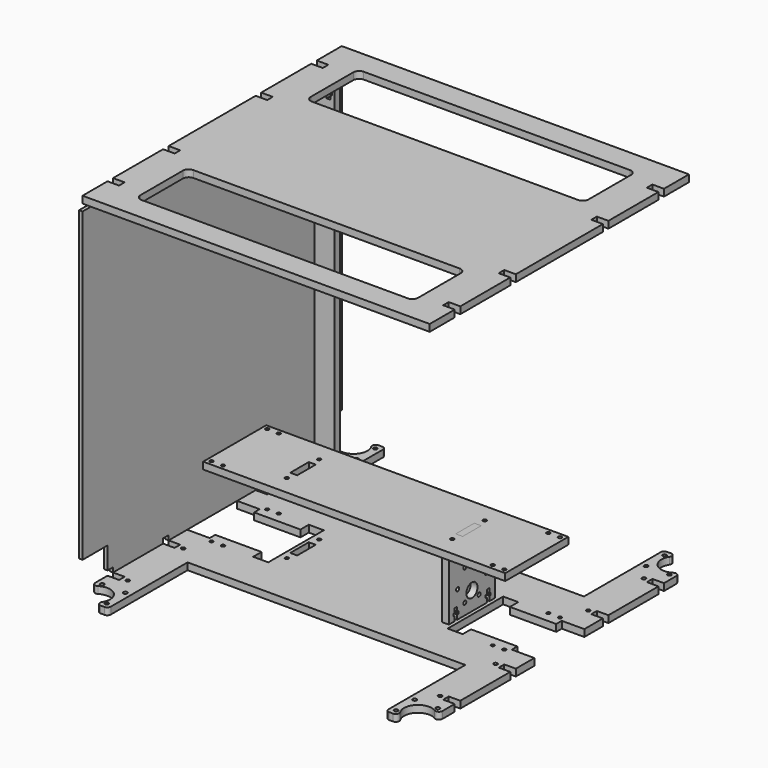
from build123d import *

# Parameters (mm, degrees)
F0_R         = 1.5
F0_W         = 6
F0_H         = 20
F1_DEPTH     = 6
F2_D         = 3
F3_W         = 6
F3_H         = 50
F4_DEPTH     = 55
F5_W         = 6
F5_H         = 20
F6_DEPTH     = 6
F7_R         = 6
F7_R_2       = 1.65
F8_DEPTH     = 6
F10_DEPTH    = 6
F11_W        = 6
F11_H        = 20
F12_DEPTH    = 6
F13_W        = 261
F13_H        = 68.1
F13_R        = 1.5
F13_W_2      = 6
F13_H_2      = 20
F14_DEPTH    = 6
F16_DEPTH    = 6
F17_W        = 10
F17_H        = 6
F19_DEPTH    = 6.001
F20_R        = 3
F21_D        = 3.3
F21_ON_F17_D = 3.3
F23_DEPTH    = 6
F25_DEPTH    = 3
F26_W        = 240
F26_H        = 55.95
F27_DEPTH    = 6
F28_R        = 5


with BuildPart() as f1:
    # F0 (on Top) → F1 (new body)
    with BuildSketch(Plane.XY):
        Polygon((150, 27), (150, 34.05), (-150, 34.05), (-150, 27), (-130.5, 27), (-130.5, 21), (-90.5, 21), (-90.5, 30), (-77.5, 30), (-77.5, -30), (-90.5, -30), (-90.5, -21), (-130.5, -21), (-130.5, -27), (-150, -27), (-150, -34.05), (150, -34.05), (150, -27), (130.5, -27), (130.5, -21), (90.5, -21), (90.5, -30), (77.5, -30), (77.5, 30), (90.5, 30), (90.5, 21), (130.5, 21), (130.5, 27), align=None)
        with Locations((-71.5, -17.5)):
            Circle(F0_R, mode=Mode.SUBTRACT)
        with Locations((71.5, -17.5)):
            Circle(F0_R, mode=Mode.SUBTRACT)
        with Locations((-71.5, 0)):
            Rectangle(F0_W, F0_H, mode=Mode.SUBTRACT)
        with Locations((-71.5, 17.5)):
            Circle(F0_R, mode=Mode.SUBTRACT)
        with Locations((71.5, 0)):
            Rectangle(F0_W, F0_H, mode=Mode.SUBTRACT)
        with Locations((71.5, 17.5)):
            Circle(F0_R, mode=Mode.SUBTRACT)
    extrude(amount=F1_DEPTH)

    # F2 (through all)
    with Locations(Plane(origin=(0, 0, 0), x_dir=(1, 0, 0), z_dir=(0, 0, -1))):
        with Locations((126.5, 30.05), (116.5, 30.05), (126.5, -30.05), (116.5, -30.05), (-116.5, 30.05), (-126.5, 30.05), (-116.5, -30.05), (-126.5, -30.05)):
            Hole(F2_D / 2)

    # F15 (on face) → F16 (join)
    with BuildSketch(Plane.XY.offset(6)):
        Polygon((-150, 150), (-150, 34.05), (0, 34.05), (150, 34.05), (150, 150), (120, 150), (120, 64.05), (0, 64.05), (-120, 64.05), (-120, 150), align=None)
        Polygon((0, -34.05), (-150, -34.05), (-150, -150), (-120, -150), (-120, -64.05), (0, -64.05), (120, -64.05), (120, -150), (150, -150), (150, -34.05), align=None)
    extrude(amount=-F16_DEPTH)

    # F17 (on face) → F19 (cut, through all)
    with BuildSketch(Plane.XY.offset(6)):
        with BuildLine():
            Line((-150, -150), (-134.2041684767, -150))
            ThreePointArc((-134.2041684767, -150), (-130.5147186258, -130.5147186258), (-150, -134.2041684767))
            Line((-150, -134.2041684767), (-150, -150))
        make_face()
        with BuildLine():
            Line((134.2041684767, -150), (150, -150))
            Line((150, -150), (150, -134.2041684767))
            ThreePointArc((150, -134.2041684767), (130.5147186258, -130.5147186258), (134.2041684767, -150))
        make_face()
        with BuildLine():
            Line((150, 150), (134.2041684767, 150))
            ThreePointArc((134.2041684767, 150), (130.5147186258, 130.5147186258), (150, 134.2041684767))
            Line((150, 134.2041684767), (150, 150))
        make_face()
        with BuildLine():
            ThreePointArc((-150, 134.2041684767), (-130.5147186258, 130.5147186258), (-134.2041684767, 150))
            Line((-134.2041684767, 150), (-150, 150))
            Line((-150, 150), (-150, 134.2041684767))
        make_face()
        with Locations((-145, 110)):
            Rectangle(F17_W, F17_H)
        with Locations((-145, 50)):
            Rectangle(F17_W, F17_H)
        with Locations((145, 50)):
            Rectangle(F17_W, F17_H)
        with Locations((145, 110)):
            Rectangle(F17_W, F17_H)
        with Locations((145, -110)):
            Rectangle(F17_W, F17_H)
        with Locations((-145, -50)):
            Rectangle(F17_W, F17_H)
        with Locations((145, -50)):
            Rectangle(F17_W, F17_H)
        with Locations((-145, -110)):
            Rectangle(F17_W, F17_H)
    extrude(amount=-F19_DEPTH, mode=Mode.SUBTRACT)

    # F20
    f20_edges = [f1.edges().sort_by_distance(p)[0] for p in [
        (-134.204168, -150, 3),
        (-150, -134.204168, 3),
        (-120, -150, 3),
        (120, -150, 3),
        (134.204168, -150, 3),
        (150, -134.204168, 3),
        (150, 134.204168, 3),
        (134.204168, 150, 3),
        (120, 150, 3),
        (-120, 150, 3),
        (-134.204168, 150, 3),
        (-150, 134.204168, 3),
    ]]
    fillet(f20_edges, radius=F20_R)

    # F21 (through all)
    with Locations(Plane.XY.offset(6)):
        with Locations((-145, 125), (-125, 145), (-125, 125), (145, 125), (125, 125), (125, 145), (-145, -125), (-125, -125), (-125, -145), (125, -145), (145, -125), (125, -125)):
            Hole(F21_D / 2)

    # F21 on F17 (through all)
    with Locations(Plane.XY.offset(6)):
        with Locations((-135, 110), (-135, 50), (-135, -50), (-135, -110), (135, -110), (135, -50), (135, 50), (135, 110)):
            Hole(F21_ON_F17_D / 2)


with BuildPart() as f4:
    # F3 (on face) → F4 (new body)
    with BuildSketch(Plane.XY.offset(6)):
        with Locations((71.5, 0)):
            Rectangle(F3_W, F3_H)
    extrude(amount=F4_DEPTH)

    # F5 (on face) → F6 (join)
    with BuildSketch(Plane(origin=(0, 0, 6), x_dir=(1, 0, 0), z_dir=(0, 0, -1))):
        with Locations((71.5, 0)):
            Rectangle(F5_W, F5_H)
    extrude(amount=F6_DEPTH)

    # F7 (on face) → F8 (cut, through all)
    with BuildSketch(Plane(origin=(68.5, 0, 0), x_dir=(0, -1, 0), z_dir=(-1, 0, 0))):
        with Locations((0, 22)):
            Circle(F7_R)
        with Locations((7.75, 15.5766062413)):
            Circle(F7_R_2)
        with Locations((15.5, 29)):
            Circle(F7_R_2)
        with Locations((7.75, 42.4233937587)):
            Circle(F7_R_2)
        with Locations((-7.75, 42.4233937587)):
            Circle(F7_R_2)
        with Locations((-15.5, 29)):
            Circle(F7_R_2)
        with Locations((-7.75, 15.5766062413)):
            Circle(F7_R_2)
    extrude(amount=-F8_DEPTH, mode=Mode.SUBTRACT)

    # F9 (on face) → F10 (cut, through all)
    with BuildSketch(Plane(origin=(68.5, 0, 0), x_dir=(0, -1, 0), z_dir=(-1, 0, 0))):
        Polygon((16, 6), (19, 6), (19, 10), (20.2, 10), (20.2, 12.3), (19, 12.3), (19, 16), (16, 16), (16, 12.3), (14.8, 12.3), (14.8, 10), (16, 10), align=None)
        Polygon((-19, 10), (-19, 6), (-16, 6), (-16, 10), (-14.8, 10), (-14.8, 12.3), (-16, 12.3), (-16, 16), (-19, 16), (-19, 12.3), (-20.2, 12.3), (-20.2, 10), align=None)
        Polygon((19, 61), (16, 61), (16, 57), (14.8, 57), (14.8, 54.7), (16, 54.7), (16, 51), (19, 51), (19, 54.7), (20.2, 54.7), (20.2, 57), (19, 57), align=None)
        Polygon((-16, 61), (-19, 61), (-19, 57), (-20.2, 57), (-20.2, 54.7), (-19, 54.7), (-19, 51), (-16, 51), (-16, 54.7), (-14.8, 54.7), (-14.8, 57), (-16, 57), align=None)
    extrude(amount=-F10_DEPTH, mode=Mode.SUBTRACT)

    # F11 (on face) → F12 (join)
    with BuildSketch(Plane.XY.offset(61)):
        with Locations((71.5, 0)):
            Rectangle(F11_W, F11_H)
    extrude(amount=F12_DEPTH)


with BuildPart() as f14:
    # F13 (on face) → F14 (new body)
    with BuildSketch(Plane.XY.offset(61)):
        Rectangle(F13_W, F13_H)
        with Locations((-126.5, -30.05)):
            Circle(F13_R, mode=Mode.SUBTRACT)
        with Locations((-116.5, -30.05)):
            Circle(F13_R, mode=Mode.SUBTRACT)
        with Locations((-71.5, -17.5)):
            Circle(F13_R, mode=Mode.SUBTRACT)
        with Locations((116.5, -30.05)):
            Circle(F13_R, mode=Mode.SUBTRACT)
        with Locations((126.5, -30.05)):
            Circle(F13_R, mode=Mode.SUBTRACT)
        with Locations((71.5, -17.5)):
            Circle(F13_R, mode=Mode.SUBTRACT)
        with Locations((-71.5, 0)):
            Rectangle(F13_W_2, F13_H_2, mode=Mode.SUBTRACT)
        with Locations((-71.5, 17.5)):
            Circle(F13_R, mode=Mode.SUBTRACT)
        with Locations((-126.5, 30.05)):
            Circle(F13_R, mode=Mode.SUBTRACT)
        with Locations((-116.5, 30.05)):
            Circle(F13_R, mode=Mode.SUBTRACT)
        with Locations((71.5, 0)):
            Rectangle(F13_W_2, F13_H_2, mode=Mode.SUBTRACT)
        with Locations((71.5, 17.5)):
            Circle(F13_R, mode=Mode.SUBTRACT)
        with Locations((116.5, 30.05)):
            Circle(F13_R, mode=Mode.SUBTRACT)
        with Locations((126.5, 30.05)):
            Circle(F13_R, mode=Mode.SUBTRACT)
    extrude(amount=F14_DEPTH)


with BuildPart() as f23:
    # F22 (on face) → F23 (new body)
    with BuildSketch(Plane.XZ.offset(-113)):
        Polygon((-150, 10), (-150, 0), (-140, 0), (-140, 6), (-136.6, 6), (-136.6, 9.75), (-137.8, 9.75), (-137.8, 12.25), (-136.6, 12.25), (-136.6, 16), (-133.4, 16), (-133.4, 12.25), (-132.2, 12.25), (-132.2, 9.75), (-133.4, 9.75), (-133.4, 6), (-130, 6), (-130, 294), (-133.4, 294), (-133.4, 290.25), (-132.2, 290.25), (-132.2, 287.75), (-133.4, 287.75), (-133.4, 284), (-136.6, 284), (-136.6, 287.75), (-137.8, 287.75), (-137.8, 290.25), (-136.6, 290.25), (-136.6, 294), (-140, 294), (-140, 300), (-150, 300), (-150, 290), (-147, 290), (-147, 10), align=None)
    extrude(amount=F23_DEPTH)


with BuildPart() as f25:
    # F24 (on face) → F25 (new body)
    with BuildSketch(Plane(origin=(-150, 0, 0), x_dir=(0, -1, 0), z_dir=(-1, 0, 0))):
        Polygon((-140, 150), (-140, 29), (-113, 29), (-113, 10), (-107, 10), (-107, 6), (-53, 6), (-53, 10), (-47, 10), (-47, 6), (47, 6), (47, 10), (53, 10), (53, 6), (107, 6), (107, 10), (113, 10), (113, 29), (140, 29), (140, 150), (140, 294), (113, 294), (113, 290), (107, 290), (107, 294), (53, 294), (53, 290), (47, 290), (47, 294), (-47, 294), (-47, 290), (-53, 290), (-53, 294), (-107, 294), (-107, 290), (-113, 290), (-113, 294), (-140, 294), align=None)
    extrude(amount=F25_DEPTH)


with BuildPart() as f27:
    # F26 (on face) → F27 (new body)
    with BuildSketch(Plane.XY.offset(300)):
        Polygon((0, 140), (-150, 140), (-150, 113), (-140, 113), (-140, 107), (-150, 107), (-150, 53), (-140, 53), (-140, 47), (-150, 47), (-150, 0), (-150, -47), (-140, -47), (-140, -53), (-150, -53), (-150, -107), (-140, -107), (-140, -113), (-150, -113), (-150, -140), (0, -140), (150, -140), (150, -113), (140, -113), (140, -107), (150, -107), (150, -53), (140, -53), (140, -47), (150, -47), (150, 0), (150, 47), (140, 47), (140, 53), (150, 53), (150, 107), (140, 107), (140, 113), (150, 113), (150, 140), align=None)
        with Locations((0, -92.025)):
            Rectangle(F26_W, F26_H, mode=Mode.SUBTRACT)
        with Locations((0, 92.025)):
            Rectangle(F26_W, F26_H, mode=Mode.SUBTRACT)
    extrude(amount=F27_DEPTH)

    # F28
    f28_edges = [f27.edges().sort_by_distance(p)[0] for p in [
        (-120, 120, 303),
        (-120, 64.05, 303),
        (120, 120, 303),
        (120, 64.05, 303),
        (120, -120, 303),
        (120, -64.05, 303),
        (-120, -64.05, 303),
        (-120, -120, 303),
    ]]
    fillet(f28_edges, radius=F28_R)


solid = Compound([f1.part, f4.part, f14.part, f23.part, f25.part, f27.part])
